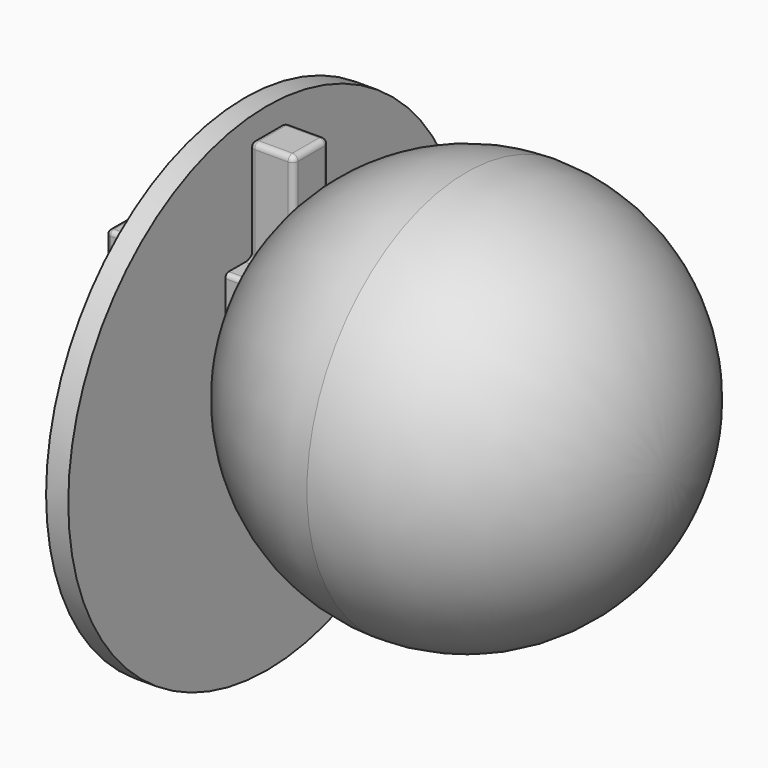
from build123d import *

# Parameters (mm, degrees)
F0_W     = 273.05
F0_H     = 119.38
F1_DEPTH = 76.2
F2_W     = 50.8
F2_H     = 50.8
F3_DEPTH = 119.38
F4_R     = 6.35
F5_R     = 5.08
F6_R     = 284.48
F6_R_2   = 38.1
F7_DEPTH = 25.4
F8_R     = 228.6
F9_DEPTH = 457.2
F10_R    = 228.59999


# Not quite as in the source:
# - a fillet or chamfer is up to 0.001 mm smaller than in the source, because OpenCascade refuses the exact size


with BuildPart() as f1:
    # F0 (on Top) → F1 (new body)
    with BuildSketch(Plane.XY):
        Rectangle(F0_W, F0_H)
    extrude(amount=F1_DEPTH)

    # F2 (on face) → F3 (join)
    with BuildSketch(Plane.XY.offset(76.2)):
        with Locations((25.4, 0)):
            Rectangle(F2_W, F2_H)
    extrude(amount=F3_DEPTH)

    # F4
    f4_edges = [f1.edges().sort_by_distance(p)[0] for p in [
        (0, 25.4, 135.89),
        (0, -25.4, 135.89),
        (0, 0, 76.2),
        (0, 0, 195.58),
        (50.8, 25.4, 135.89),
        (25.4, 25.4, 76.2),
        (25.4, 25.4, 195.58),
        (50.8, -25.4, 135.89),
        (50.8, 0, 76.2),
        (50.8, 0, 195.58),
        (25.4, -25.4, 76.2),
        (25.4, -25.4, 195.58),
    ]]
    fillet(f4_edges, radius=F4_R)

    # F5
    f5_edges = [f1.edges().sort_by_distance(p)[0] for p in [
        (-6.35, 0, 76.2),
        (-2.630256, 28.030256, 76.2),
        (-2.630256, -28.030256, 76.2),
        (25.4, 31.75, 76.2),
        (25.4, -31.75, 76.2),
        (53.430256, 28.030256, 76.2),
        (53.430256, -28.030256, 76.2),
        (57.15, 0, 76.2),
        (0, 59.69, 76.2),
        (136.525, 0, 76.2),
        (-136.525, 0, 76.2),
        (0, -59.69, 76.2),
        (0, 59.69, 0),
        (-136.525, 0, 0),
        (0, -59.69, 0),
        (136.525, 0, 0),
        (-136.525, -59.69, 38.1),
        (136.525, -59.69, 38.1),
        (136.525, 59.69, 38.1),
        (-136.525, 59.69, 38.1),
    ]]
    fillet(f5_edges, radius=F5_R)


with BuildPart() as f7:
    # F6 (on Right) → F7 (new body)
    with BuildSketch(Plane.YZ):
        with Locations((0, -63.5)):
            Circle(F6_R)
        with Locations((0, -63.5)):
            Circle(F6_R_2, mode=Mode.SUBTRACT)
    extrude(amount=-F7_DEPTH)


with BuildPart() as f9:
    # F8 (on Right) → F9 (new body)
    with BuildSketch(Plane.YZ):
        Circle(F8_R)
    extrude(amount=F9_DEPTH)

    # F10 (radius 228.6 in the source; OpenCascade refuses exactly that, so slightly less here)
    f10_edges = [f9.edges().sort_by_distance(p)[0] for p in [
        (457.2, -228.6, 0),
        (0, -228.6, 0),
    ]]
    fillet(f10_edges, radius=F10_R)


solid = Compound([f1.part, f7.part, f9.part])
